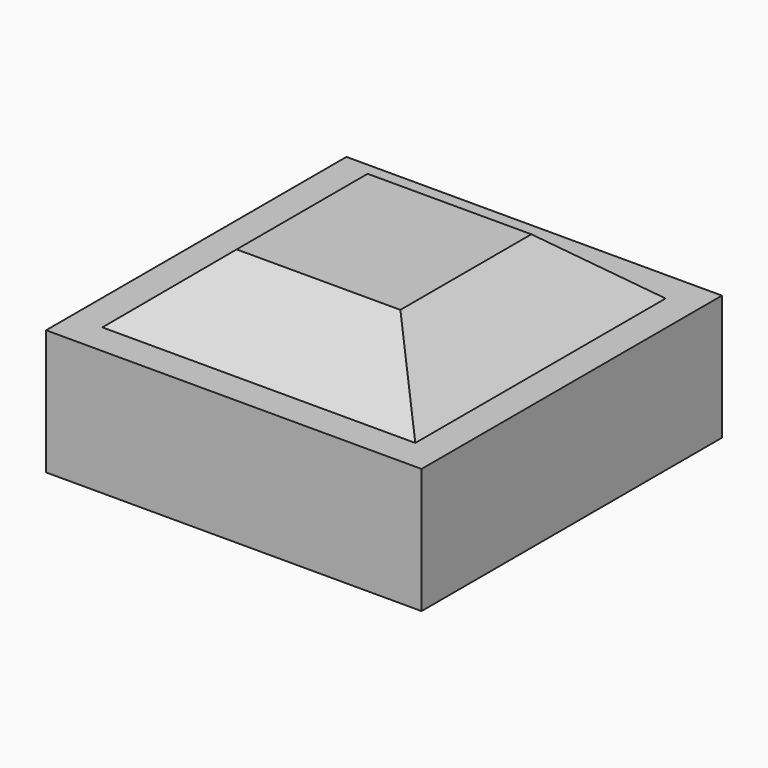
from build123d import *

# Parameters (mm, degrees)
F0_W     = 76.2
F0_H     = 76.2
F1_DEPTH = 25.4
F2_W     = 63.5
F2_H     = 63.5
F3_DEPTH = 12.7
F4_SIZE2 = 15.135261
F4_SIZE  = 12.69999


# Not quite as in the source:
# - a fillet or chamfer is up to 0.001 mm smaller than in the source, because OpenCascade refuses the exact size


with BuildPart() as f1:
    # F0 (on Top) → F1 (new body)
    with BuildSketch(Plane.XY):
        Rectangle(F0_W, F0_H)
    extrude(amount=F1_DEPTH)

    # F2 (on face) → F3 (join)
    with BuildSketch(Plane.XY.offset(25.4)):
        Rectangle(F2_W, F2_H)
    extrude(amount=F3_DEPTH)

    # F4 (size 12.7 and 15.1352706259 in the source; OpenCascade refuses exactly that, so slightly less here)
    f4_edges = [f1.edges().sort_by_distance(p)[0] for p in [
        (0, -31.75, 38.1),
        (-31.75, 0, 38.1),
        (0, 31.75, 38.1),
        (31.75, 0, 38.1),
    ]]
    chamfer(f4_edges, length=F4_SIZE, length2=F4_SIZE2)


solid = f1.part
